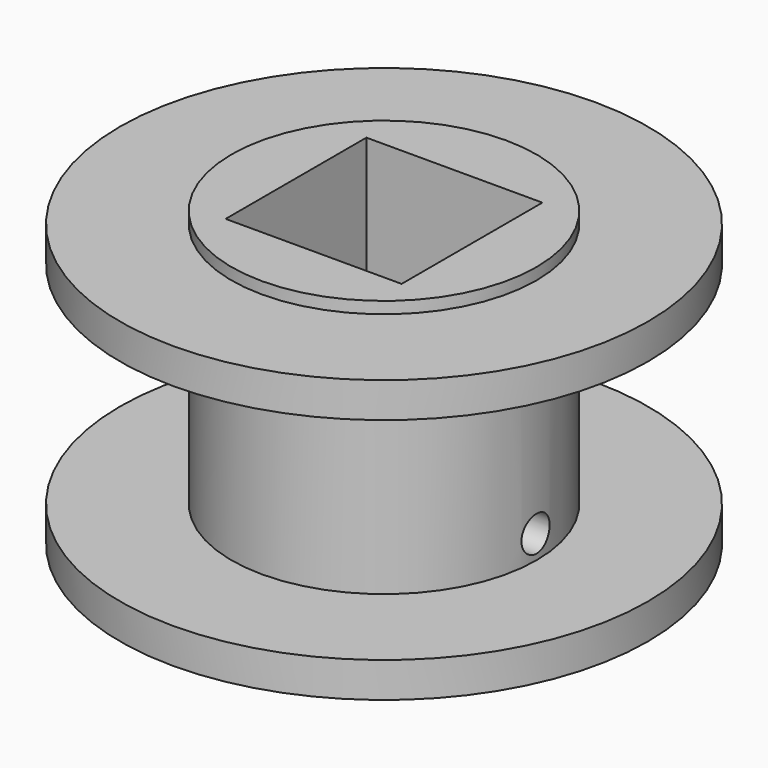
from build123d import *

# Parameters (mm, degrees)
F0_R     = 13
F1_DEPTH = 13
F3_R     = 22.5
F4_DEPTH = 3
F5_W     = 15
F5_H     = 15
F6_DEPTH = 58.6
F7_R     = 1.5
F8_DEPTH = 25


# Not quite as in the source:
# - a pattern or mirror of a feature is missing from the dataset's text; its kind, count and spacing are read off the source's solid


with BuildPart() as f1:
    # F0 (on Top) → F1 (new body, symmetric)
    with BuildSketch(Plane.XY):
        Circle(F0_R)
    extrude(amount=F1_DEPTH, both=True)

    # F3 (on offset) → F4 (join)
    with BuildSketch(Plane.XY.offset(12)):
        Circle(F3_R)
    f4 = extrude(amount=-F4_DEPTH)

    # F4_copies: F4 across plane
    add(f4.mirror(Plane(origin=(0, 0, 0), x_dir=(-1, 0, 0), z_dir=(0, 0, -1))))

    # F5 (on face) → F6 (cut)
    with BuildSketch(Plane.XY.offset(13)):
        Rectangle(F5_W, F5_H)
    extrude(amount=-F6_DEPTH, mode=Mode.SUBTRACT)

    # F7 (on Right) → F8 (cut, symmetric)
    with BuildSketch(Plane.YZ):
        with Locations((0, -7)):
            Circle(F7_R)
    extrude(amount=F8_DEPTH, both=True, mode=Mode.SUBTRACT)


solid = f1.part
